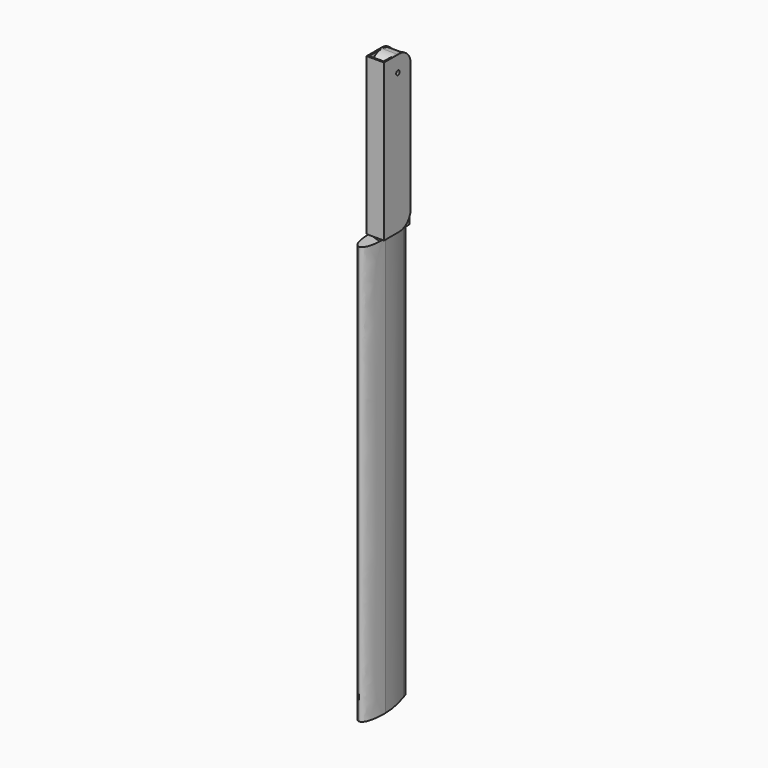
from build123d import *

# Parameters (mm, degrees)
F1_DEPTH      = 304.8
F1_DEPTH_BACK = 38.1
F2_R          = 31.75
F3_R          = 4.7625
F4_DEPTH      = 31.75
F6_DEPTH      = 914.4
F7_DEPTH      = 50.8


with BuildPart() as f1:
    # F0 (on Top) → F1 (new body, two sides)
    with BuildSketch(Plane.XY) as f1_sk:
        Polygon((-15.875, 34.925), (-19.05, 34.925), (-19.05, -38.1), (19.05, -38.1), (19.05, 34.925), (15.875, 34.925), (15.875, -34.925), (-15.875, -34.925), align=None)
    extrude(amount=-F1_DEPTH)
    extrude(f1_sk.sketch, amount=F1_DEPTH_BACK)

    # F2
    f2_edges = [f1.edges().sort_by_distance(p)[0] for p in [
        (-17.4625, 34.925, 38.1),
        (17.4625, 34.925, 38.1),
        (-17.4625, 34.925, -304.8),
        (17.4625, 34.925, -304.8),
    ]]
    fillet(f2_edges, radius=F2_R)

    # F3 (on face) → F7 (cut, symmetric)
    with BuildSketch(Plane.YZ.offset(-15.875)):
        with Locations((0, 3.0427083333)):
            Circle(F3_R)
    extrude(amount=F7_DEPTH, both=True, mode=Mode.SUBTRACT)


with BuildPart() as f4:
    # F3 (on face) → F4 (new body, through all)
    with BuildSketch(Plane.YZ.offset(-15.875)):
        with BuildLine():
            Line((34.925, -273.05), (34.925, 0))
            Line((34.925, 0), (34.925, 6.0854166667))
            ThreePointArc((34.925, 6.0854166667), (23.6890754365, 28.8853359855), (1.308e-07, 38.1))
            ThreePointArc((1.308e-07, 38.1), (-23.6890753401, 28.8853360738), (-34.925, 6.0854166667))
            Line((-34.925, 6.0854166667), (-34.925, 0))
            Line((-34.925, 0), (-34.925, -304.8))
            Line((-34.925, -304.8), (3.175, -304.8))
            ThreePointArc((3.175, -304.8), (25.6256403027, -295.5006403027), (34.925, -273.05))
        make_face()
        with Locations((0, 3.0427083333)):
            Circle(F3_R, mode=Mode.SUBTRACT)
        with BuildLine():
            Line((34.925, -304.8), (34.925, -273.05))
            ThreePointArc((34.925, -273.05), (25.6256403027, -295.5006403027), (3.175, -304.8))
            Line((3.175, -304.8), (34.925, -304.8))
        make_face()
    extrude(amount=F4_DEPTH)

    # F5 (on face) → F6 (join)
    with BuildSketch(Plane(origin=(0, 0, -304.8), x_dir=(1, 0, 0), z_dir=(0, 0, -1))):
        with BuildLine():
            add(Edge.make_bspline(
                [(0, 82.55), (12.0985200629, 82.6351493597), (16.314810061, 53.6201264646), (15.875, 29.9038812518)],
                knots=[0, 0, 0, 0, 0.4595861737, 0.4595861737, 0.4595861737, 0.4595861737], degree=3))
            add(Edge.make_bspline(
                [(0, 82.55), (-12.0985200629, 82.6351493597), (-16.314810061, 53.6201264646), (-15.875, 29.9038812518)],
                knots=[0, 0, 0, 0, 0.4595861737, 0.4595861737, 0.4595861737, 0.4595861737], degree=3))
            Line((-15.875, 29.9038812518), (-15.875, 34.925))
            Line((-15.875, 34.925), (15.875, 34.925))
            Line((15.875, 34.925), (15.875, 29.9038812518))
        make_face()
        with BuildLine():
            add(Edge.make_bspline(
                [(15.875, 29.9038812518), (15.4227365407, 5.516101041), (10.0469612559, -13.2685790973), (3.0850515824, -34.925)],
                knots=[0.4595861737, 0.4595861737, 0.4595861737, 0.4595861737, 0.9321857143, 0.9321857143, 0.9321857143, 0.9321857143], degree=3))
            Line((15.875, 29.9038812518), (15.875, 34.925))
            Line((15.875, 34.925), (-15.875, 34.925))
            Line((-15.875, 34.925), (-15.875, 29.9038812518))
            add(Edge.make_bspline(
                [(-15.875, 29.9038812518), (-15.4227365407, 5.516101041), (-10.0469612559, -13.2685790973), (-3.0850515824, -34.925)],
                knots=[0.4595861737, 0.4595861737, 0.4595861737, 0.4595861737, 0.9321857143, 0.9321857143, 0.9321857143, 0.9321857143], degree=3))
            Line((-3.0850515824, -34.925), (3.0850515824, -34.925))
        make_face()
        with BuildLine():
            add(Edge.make_bspline(
                [(3.0850515824, -34.925), (2.0860727621, -38.0325246332), (1.0544354764, -41.1991783333), (0, -44.45)],
                knots=[0.9321857143, 0.9321857143, 0.9321857143, 0.9321857143, 1, 1, 1, 1], degree=3))
            Line((3.0850515824, -34.925), (-3.0850515824, -34.925))
            add(Edge.make_bspline(
                [(-3.0850515824, -34.925), (-2.0860727621, -38.0325246332), (-1.0544354764, -41.1991783333), (0, -44.45)],
                knots=[0.9321857143, 0.9321857143, 0.9321857143, 0.9321857143, 1, 1, 1, 1], degree=3))
        make_face()
    extrude(amount=F6_DEPTH)


solid = Compound([f1.part, f4.part])
